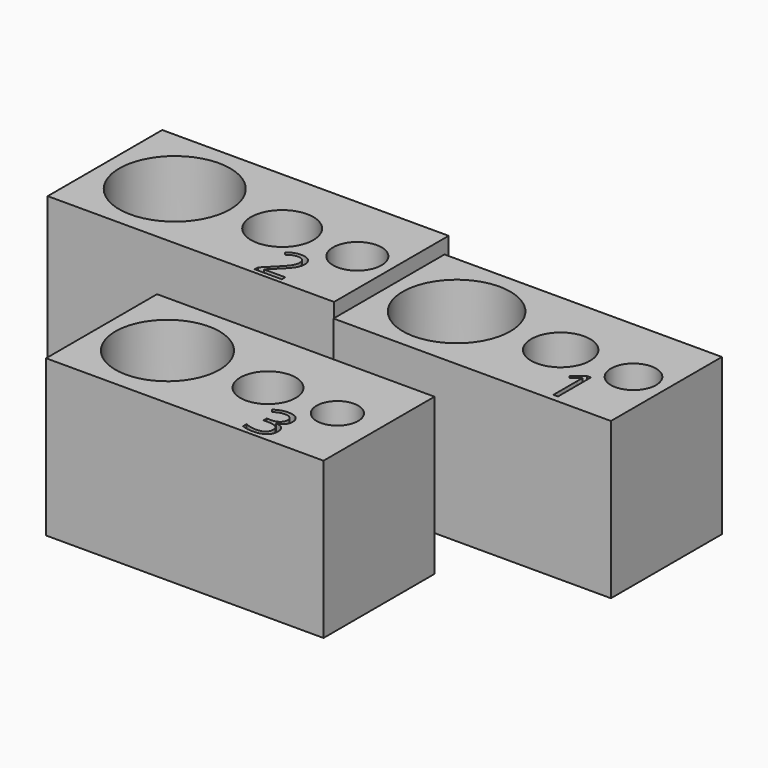
from build123d import *

# Parameters (mm, degrees)
F1_W         = 82.5806451613
F1_H         = 41.2903225806
F1_R         = 16
F1_R_2       = 7
F1_R_3       = 9
F3_DEPTH     = 45
F0_W         = 80
F0_H         = 40
F0_R         = 15.5
F0_R_2       = 8.5
F0_R_3       = 6.5
F2_W         = 80
F2_H         = 40
F2_R         = 15
F2_R_2       = 8
F2_R_3       = 6
F4_TEXT_SIZE = 16.6666666667
F5_DEPTH     = 5


# Not quite as in the source:
# - Text() gives the source's letters only with a copy of the font that has no kerning and outlines rounded to 1/6400 em; it was checked with that copy


with BuildPart() as f3:
    # F1 (on Top) → F3 (new body)
    with BuildSketch(Plane.XY):
        with Locations((-46.4857211709, 28.1999981776)):
            Rectangle(F1_W, F1_H)
        with Locations((-67.6470114935, 28.1999981776)):
            Circle(F1_R, mode=Mode.SUBTRACT)
        with Locations((-15.0018502032, 28.1999981776)):
            Circle(F1_R_2, mode=Mode.SUBTRACT)
        with Locations((-36.679269558, 28.1999981776)):
            Circle(F1_R_3, mode=Mode.SUBTRACT)
    extrude(amount=F3_DEPTH)


with BuildPart() as f3b:
    # F0 (on Top) → F3, piece 2 (new body)
    with BuildSketch(Plane.XY):
        with Locations((39.7537503533, 21.1563933532)):
            Rectangle(F0_W, F0_H)
        with Locations((19.2537503533, 21.1563933532)):
            Circle(F0_R, mode=Mode.SUBTRACT)
        with Locations((49.2537503533, 21.1563933532)):
            Circle(F0_R_2, mode=Mode.SUBTRACT)
        with Locations((70.2537503533, 21.1563933532)):
            Circle(F0_R_3, mode=Mode.SUBTRACT)
    extrude(amount=F3_DEPTH)


with BuildPart() as f3c:
    # F2 (on Top) → F3, piece 3 (new body)
    with BuildSketch(Plane.XY):
        with Locations((1.3228812814, -34.3988868594)):
            Rectangle(F2_W, F2_H)
        with Locations((-19.6771187186, -34.3988868594)):
            Circle(F2_R, mode=Mode.SUBTRACT)
        with Locations((9.3228812814, -34.3988868594)):
            Circle(F2_R_2, mode=Mode.SUBTRACT)
        with Locations((29.3228812814, -34.3988868594)):
            Circle(F2_R_3, mode=Mode.SUBTRACT)
    extrude(amount=F3_DEPTH)


with BuildPart() as f5_tool:
    # F4 (on face) → F5 (new body)
    with BuildSketch(Plane.XY.offset(45)):
        with Locations((57.1597545939, 3.0313965638)):
            Text('1', F4_TEXT_SIZE, font='Open Sans', text_align=(TextAlign.LEFT, TextAlign.BOTTOM))
        with Locations((-29.9098998273, 8.8152978569)):
            Text('2', F4_TEXT_SIZE, font='Open Sans', text_align=(TextAlign.LEFT, TextAlign.BOTTOM))
        with Locations((15.8836204792, -53.0205237567)):
            Text('3', F4_TEXT_SIZE, font='Open Sans', text_align=(TextAlign.LEFT, TextAlign.BOTTOM))
    extrude(amount=-F5_DEPTH)


with BuildPart() as f3_1:
    add(f3.part)

    # F5: cut by f5_tool
    add(f5_tool.part, mode=Mode.SUBTRACT)


with BuildPart() as f3b_1:
    add(f3b.part)

    # F5: cut by f5_tool
    add(f5_tool.part, mode=Mode.SUBTRACT)


with BuildPart() as f3c_1:
    add(f3c.part)

    # F5: cut by f5_tool
    add(f5_tool.part, mode=Mode.SUBTRACT)


solid = Compound([f3_1.part, f3b_1.part, f3c_1.part])
